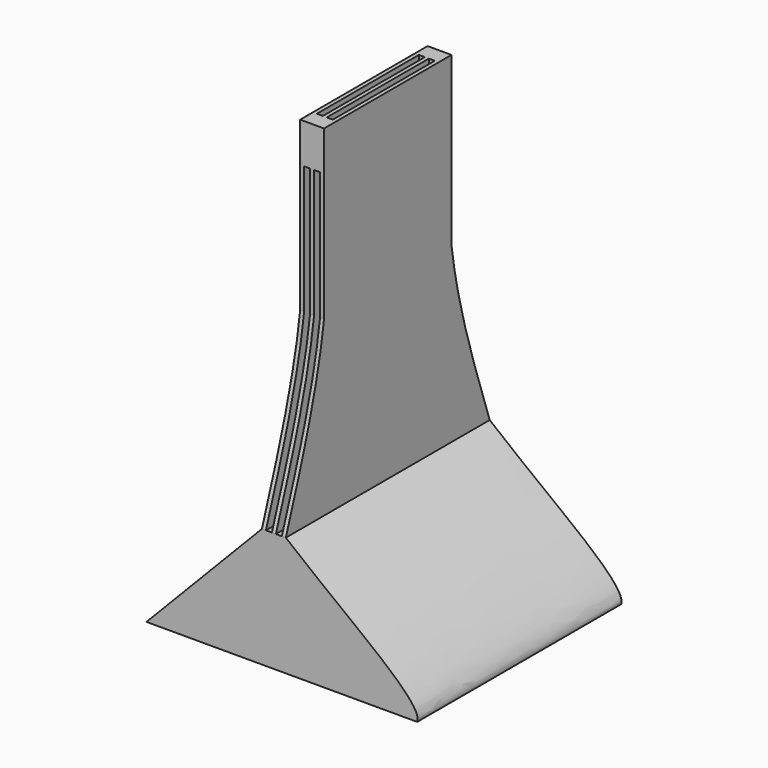
from build123d import *

# Parameters (mm, degrees)
F1_DEPTH  = 320
F2_W      = 30
F2_H      = 320
F3_DEPTH  = 428
F5_DEPTH  = 205
F7_W      = 260
F7_H      = 128.6325914682
F8_DEPTH  = 30
F9_W      = 7.5
F9_H      = 457.219858036
F10_DEPTH = 977
F6_W      = 20
F6_H      = 50
F6_H_2    = 25
F11_DEPTH = 25
F12_R     = 5.1978686685
F13_DEPTH = 63


with BuildPart() as f1:
    # F0 (on Front) → F1 (new body)
    with BuildSketch(Plane.XZ):
        with BuildLine():
            Line((150.299176857, 1.1440683747), (180.299176857, 1.1440683747))
            Line((180.299176857, 1.1440683747), (340.299176857, 1.1440683747))
            add(Edge.make_bspline(
                [(340.299176857, 1.1440683747), (349.1569172885, 24.1151609846), (251.1032390966, 88.0444564268), (175.3079980464, 151.1440683747)],
                knots=[0.4586039165, 0.4586039165, 0.4586039165, 0.4586039165, 1, 1, 1, 1], degree=3))
            Line((175.3079980464, 151.1440683747), (145.3079980464, 151.1440683747))
            Line((145.3079980464, 151.1440683747), (0.299176857, 1.1440683747))
            Line((0.299176857, 1.1440683747), (100.299176857, 1.1440683747))
            Line((100.299176857, 1.1440683747), (150.299176857, 1.1440683747))
        make_face()
    extrude(amount=F1_DEPTH)

    # F2 (on face) → F3 (join)
    with BuildSketch(Plane.XY.offset(151.1440683747)):
        with Locations((160.3079980464, -160)):
            Rectangle(F2_W, F2_H)
    extrude(amount=F3_DEPTH)

    # F4 (on face) → F5 (cut)
    with BuildSketch(Plane(origin=(145.3079980464, 0, 0), x_dir=(0, -1, 0), z_dir=(-1, 0, 0))):
        with BuildLine():
            Line((0, 579.1440683747), (0, 151.1440683747))
            add(Edge.make_bspline(
                [(60, 368.6685562134), (50.1739969339, 296.0916949665), (25.086998467, 223.6178816706), (0, 151.1440683747)],
                knots=[0.4913001533, 0.4913001533, 0.4913001533, 0.4913001533, 1, 1, 1, 1], degree=3))
            Line((60, 368.6685562134), (60, 579.1440683747))
            Line((60, 579.1440683747), (0, 579.1440683747))
        make_face()
        with BuildLine():
            add(Edge.make_bspline(
                [(320, 151.1440683747), (294.913001533, 223.6178816706), (269.8260030661, 296.0916949665), (260, 368.6685562134)],
                knots=[0, 0, 0, 0, 0.5086998467, 0.5086998467, 0.5086998467, 0.5086998467], degree=3))
            Line((320, 151.1440683747), (320, 579.1440683747))
            Line((320, 579.1440683747), (260, 579.1440683747))
            Line((260, 579.1440683747), (260, 368.6685562134))
        make_face()
    extrude(amount=-F5_DEPTH, mode=Mode.SUBTRACT)

    # F7 (on face) → F8 (cut)
    with BuildSketch(Plane(origin=(-0.4170581217, 0, 0.4031807106), x_dir=(0, -1, 0), z_dir=(-0.7189672474, 0, 0.6950439534))):
        with Locations((160, 105.3467844897)):
            Rectangle(F7_W, F7_H)
    extrude(amount=-F8_DEPTH, mode=Mode.SUBTRACT)

    # F9 (on face) → F10 (cut)
    with BuildSketch(Plane.XZ.offset(320)):
        with Locations((154.0579980464, 379.7539973927)):
            Rectangle(F9_W, F9_H)
        with Locations((166.5579980464, 379.7539973927)):
            Rectangle(F9_W, F9_H)
    extrude(amount=-F10_DEPTH, mode=Mode.SUBTRACT)

    # F6 (on face) → F11 (join)
    with BuildSketch(Plane.YZ.offset(175.3079980464)):
        with Locations((-250, 554.1440683747)):
            Rectangle(F6_W, F6_H)
        with Locations((-70, 554.1440683747)):
            Rectangle(F6_W, F6_H)
        with Locations((-230, 406.1685562134)):
            Rectangle(F6_W, F6_H_2)
        with Locations((-90, 406.1685562134)):
            Rectangle(F6_W, F6_H_2)
    extrude(amount=-F11_DEPTH)

    # F12 (on Right) → F13 (cut)
    with BuildSketch(Plane.YZ):
        with Locations((-268.3978974819, 7.7915792353)):
            Circle(F12_R)
    extrude(amount=F13_DEPTH, mode=Mode.SUBTRACT)


solid = f1.part
